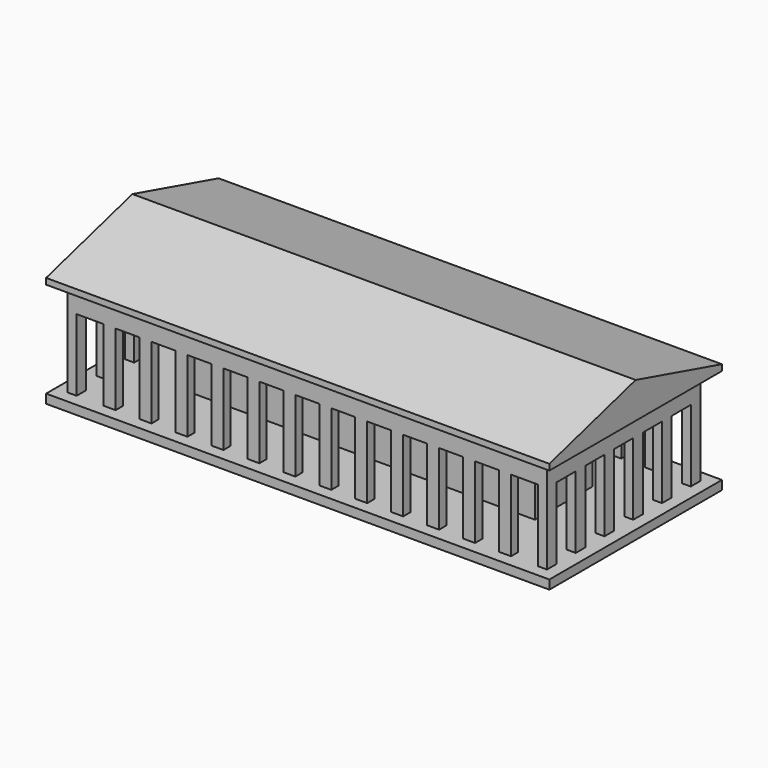
from build123d import *

# Parameters (mm, degrees)
F0_W     = 266.7
F0_H     = 114.3
F1_DEPTH = 4.7625
F2_W     = 4.7625
F2_H     = 6.35
F2_W_2   = 6.35
F2_H_2   = 4.7625
F3_DEPTH = 38.1
F4_W     = 190.5
F4_H     = 38.1
F4_W_2   = 180.975
F4_H_2   = 28.575
F5_DEPTH = 50.8
F6_W     = 4.7625
F6_H     = 6.35
F7_DEPTH = 12.7
F9_DEPTH = 266.7


# Not quite as in the source:
# - a feature names something its author has since deleted; it is built from what else it names


with BuildPart() as f1:
    # F0 (on Top) → F1 (new body)
    with BuildSketch(Plane.XY):
        Rectangle(F0_W, F0_H)
    extrude(amount=F1_DEPTH)

    # F2 (on face) → F3 (join)
    with BuildSketch(Plane.XY.offset(4.7625)):
        with Locations((-124.61875, -47.625)):
            Rectangle(F2_W, F2_H)
        with Locations((-124.61875, -9.525)):
            Rectangle(F2_W, F2_H)
        with Locations((-124.61875, 9.525)):
            Rectangle(F2_W, F2_H)
        with Locations((-124.61875, 28.575)):
            Rectangle(F2_W, F2_H)
        with Locations((-124.61875, 47.625)):
            Rectangle(F2_W, F2_H)
        with Locations((124.61875, 47.625)):
            Rectangle(F2_W, F2_H)
        with Locations((124.61875, -47.625)):
            Rectangle(F2_W, F2_H)
        with Locations((124.61875, 28.575)):
            Rectangle(F2_W, F2_H)
        with Locations((124.61875, 9.525)):
            Rectangle(F2_W, F2_H)
        with Locations((124.61875, -9.525)):
            Rectangle(F2_W, F2_H)
        with Locations((124.61875, -28.575)):
            Rectangle(F2_W, F2_H)
        with Locations((-104.775, 48.41875)):
            Rectangle(F2_W_2, F2_H_2)
        with Locations((-85.725, 48.41875)):
            Rectangle(F2_W_2, F2_H_2)
        with Locations((-66.675, 48.41875)):
            Rectangle(F2_W_2, F2_H_2)
        with Locations((-47.625, 48.41875)):
            Rectangle(F2_W_2, F2_H_2)
        with Locations((-28.575, 48.41875)):
            Rectangle(F2_W_2, F2_H_2)
        with Locations((-9.525, 48.41875)):
            Rectangle(F2_W_2, F2_H_2)
        with Locations((9.525, 48.41875)):
            Rectangle(F2_W_2, F2_H_2)
        with Locations((28.575, 48.41875)):
            Rectangle(F2_W_2, F2_H_2)
        with Locations((47.625, 48.41875)):
            Rectangle(F2_W_2, F2_H_2)
        with Locations((66.675, 48.41875)):
            Rectangle(F2_W_2, F2_H_2)
        with Locations((85.725, 48.41875)):
            Rectangle(F2_W_2, F2_H_2)
        with Locations((104.775, 48.41875)):
            Rectangle(F2_W_2, F2_H_2)
        with Locations((-124.61875, -28.575)):
            Rectangle(F2_W, F2_H)
        with Locations((-85.725, -48.41875)):
            Rectangle(F2_W_2, F2_H_2)
        with Locations((-104.775, -48.41875)):
            Rectangle(F2_W_2, F2_H_2)
        with Locations((-66.675, -48.41875)):
            Rectangle(F2_W_2, F2_H_2)
        with Locations((-47.625, -48.41875)):
            Rectangle(F2_W_2, F2_H_2)
        with Locations((-28.575, -48.41875)):
            Rectangle(F2_W_2, F2_H_2)
        with Locations((-9.525, -48.41875)):
            Rectangle(F2_W_2, F2_H_2)
        with Locations((9.525, -48.41875)):
            Rectangle(F2_W_2, F2_H_2)
        with Locations((28.575, -48.41875)):
            Rectangle(F2_W_2, F2_H_2)
        with Locations((47.625, -48.41875)):
            Rectangle(F2_W_2, F2_H_2)
        with Locations((66.675, -48.41875)):
            Rectangle(F2_W_2, F2_H_2)
        with Locations((85.725, -48.41875)):
            Rectangle(F2_W_2, F2_H_2)
        with Locations((104.775, -48.41875)):
            Rectangle(F2_W_2, F2_H_2)
    extrude(amount=F3_DEPTH)

    # F4 (on face) → F5 (join)
    with BuildSketch(Plane.XY.offset(4.7625)):
        Rectangle(F4_W, F4_H)
        Rectangle(F4_W_2, F4_H_2, mode=Mode.SUBTRACT)
    extrude(amount=F5_DEPTH)

    # F6 (on face) → F7 (join)
    with BuildSketch(Plane.XY.offset(42.8625)):
        Polygon((127, 50.8), (-127, 50.8), (-127, 31.75), (-122.2375, 31.75), (-122.2375, 46.0375), (122.2375, 46.0375), (122.2375, -46.0375), (-122.2375, -46.0375), (-122.2375, 25.4), (-127, 25.4), (-127, -50.8), (127, -50.8), align=None)
        with Locations((-124.61875, 28.575)):
            Rectangle(F6_W, F6_H)
    extrude(amount=F7_DEPTH)

    # F8 (on face) → F9 (join, through all)
    with BuildSketch(Plane(origin=(-133.35, 0, 0), x_dir=(0, -1, 0), z_dir=(-1, 0, 0))):
        Polygon((-57.15, 55.5625), (-50.8, 55.5625), (50.8, 55.5625), (57.15, 55.5625), (57.15, 58.7375), (0, 74.6125), (-57.15, 58.7375), align=None)
    extrude(amount=-F9_DEPTH)


solid = f1.part
